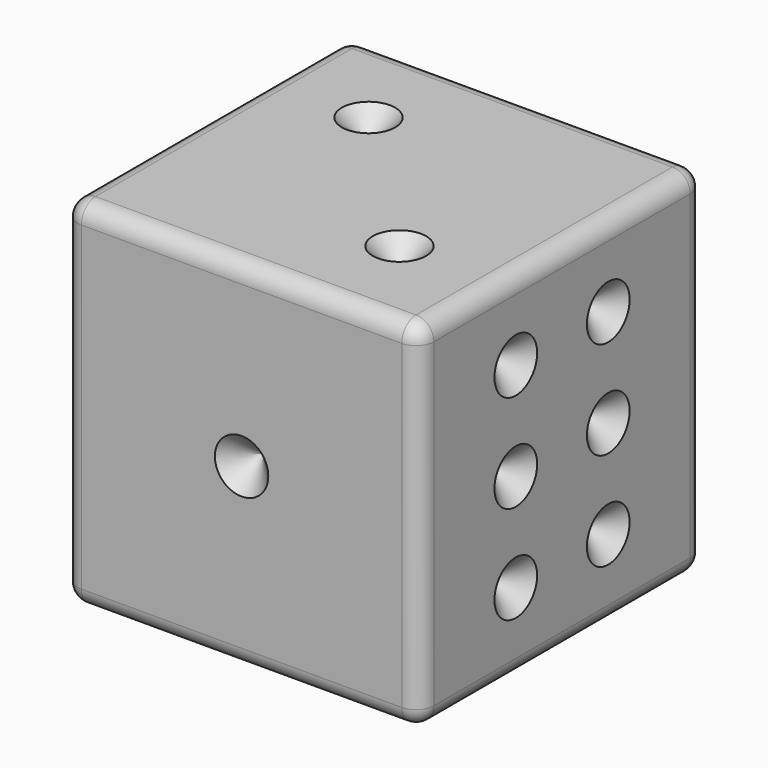
from build123d import *

# Parameters (mm, degrees)
F0_W      = 20
F0_H      = 20
F1_DEPTH  = 20
F2_R      = 1.5
F3_DEPTH  = 1.5
F4_R      = 1.5
F5_DEPTH  = 1.5
F6_SIZE   = 1.49999
F7_SIZE   = 1.49999
F8_R      = 1.5
F9_DEPTH  = 1.5
F10_SIZE  = 1.49999
F11_R     = 1.5
F12_DEPTH = 1.5
F13_SIZE  = 1.49999
F14_R     = 1.5
F15_DEPTH = 1.5
F16_SIZE  = 1.49999
F17_R     = 1.5
F18_DEPTH = 1.5
F19_SIZE  = 1.49999
F20_R     = 1


# Not quite as in the source:
# - a fillet or chamfer is up to 0.001 mm smaller than in the source, because OpenCascade refuses the exact size


with BuildPart() as f1:
    # F0 (on Top) → F1 (new body)
    with BuildSketch(Plane.XY):
        with Locations((10, 10)):
            Rectangle(F0_W, F0_H)
    extrude(amount=F1_DEPTH)

    # F2 (on face) → F3 (cut)
    with BuildSketch(Plane.XZ):
        with Locations((10, 10)):
            Circle(F2_R)
    extrude(amount=-F3_DEPTH, mode=Mode.SUBTRACT)

    # F4 (on face) → F5 (cut)
    with BuildSketch(Plane.XY.offset(20)):
        with Locations((5.6568542495, 14.3431457505)):
            Circle(F4_R)
        with Locations((14.3431457505, 5.6568542495)):
            Circle(F4_R)
    extrude(amount=-F5_DEPTH, mode=Mode.SUBTRACT)

    # F6 (size 1.5 in the source; OpenCascade refuses exactly that, so slightly less here)
    f6_edges = [f1.edges().sort_by_distance(p)[0] for p in [
        (12.843146, 5.656854, 18.5),
        (4.156854, 14.343146, 18.5),
    ]]
    chamfer(f6_edges, length=F6_SIZE)

    # F7 (size 1.5 in the source; OpenCascade refuses exactly that, so slightly less here)
    f7_edges = [f1.edges().sort_by_distance(p)[0] for p in [
        (8.5, 1.5, 10),
    ]]
    chamfer(f7_edges, length=F7_SIZE)

    # F8 (on face) → F9 (cut)
    with BuildSketch(Plane(origin=(0, 20, 0), x_dir=(-1, 0, 0), z_dir=(0, 1, 0))):
        with Locations((-16.1109127035, 16.1109127035)):
            Circle(F8_R)
        with Locations((-10, 10)):
            Circle(F8_R)
        with Locations((-3.8890872965, 3.8890872965)):
            Circle(F8_R)
    extrude(amount=-F9_DEPTH, mode=Mode.SUBTRACT)

    # F10 (size 1.5 in the source; OpenCascade refuses exactly that, so slightly less here)
    f10_edges = [f1.edges().sort_by_distance(p)[0] for p in [
        (17.610913, 18.5, 16.110913),
        (11.5, 18.5, 10),
        (5.389087, 18.5, 3.889087),
    ]]
    chamfer(f10_edges, length=F10_SIZE)

    # F11 (on face) → F12 (cut)
    with BuildSketch(Plane(origin=(0, 0, 0), x_dir=(1, 0, 0), z_dir=(0, 0, -1))):
        with Locations((5.6568542495, -5.6568542495)):
            Circle(F11_R)
        with Locations((14.3431457505, -5.6568542495)):
            Circle(F11_R)
        with Locations((14.3431457505, -14.3431457505)):
            Circle(F11_R)
        with Locations((5.6568542495, -14.3431457505)):
            Circle(F11_R)
    extrude(amount=-F12_DEPTH, mode=Mode.SUBTRACT)

    # F13 (size 1.5 in the source; OpenCascade refuses exactly that, so slightly less here)
    f13_edges = [f1.edges().sort_by_distance(p)[0] for p in [
        (4.156854, 14.343146, 1.5),
        (4.156854, 5.656854, 1.5),
        (12.843146, 5.656854, 1.5),
        (12.843146, 14.343146, 1.5),
    ]]
    chamfer(f13_edges, length=F13_SIZE)

    # F14 (on face) → F15 (cut)
    with BuildSketch(Plane(origin=(0, 0, 0), x_dir=(0, -1, 0), z_dir=(-1, 0, 0))):
        with Locations((-16.1109127035, 16.1109127035)):
            Circle(F14_R)
        with Locations((-3.8890872965, 16.1109127035)):
            Circle(F14_R)
        with Locations((-10, 10)):
            Circle(F14_R)
        with Locations((-16.1109127035, 3.8890872965)):
            Circle(F14_R)
        with Locations((-3.8890872965, 3.8890872965)):
            Circle(F14_R)
    extrude(amount=-F15_DEPTH, mode=Mode.SUBTRACT)

    # F16 (size 1.5 in the source; OpenCascade refuses exactly that, so slightly less here)
    f16_edges = [f1.edges().sort_by_distance(p)[0] for p in [
        (1.5, 17.610913, 16.110913),
        (1.5, 5.389087, 16.110913),
        (1.5, 11.5, 10),
        (1.5, 5.389087, 3.889087),
        (1.5, 17.610913, 3.889087),
    ]]
    chamfer(f16_edges, length=F16_SIZE)

    # F17 (on face) → F18 (cut)
    with BuildSketch(Plane.YZ.offset(20)):
        with Locations((6.7543126643, 15.5)):
            Circle(F17_R)
        with Locations((13.246, 4.5)):
            Circle(F17_R)
        with Locations((6.7543126643, 4.5)):
            Circle(F17_R)
        with Locations((13.246, 15.5)):
            Circle(F17_R)
        with Locations((13.246, 10)):
            Circle(F17_R)
        with Locations((6.7543126643, 10)):
            Circle(F17_R)
    extrude(amount=-F18_DEPTH, mode=Mode.SUBTRACT)

    # F19 (size 1.5 in the source; OpenCascade refuses exactly that, so slightly less here)
    f19_edges = [f1.edges().sort_by_distance(p)[0] for p in [
        (18.5, 5.254313, 15.5),
        (18.5, 11.746, 15.5),
        (18.5, 5.254313, 10),
        (18.5, 11.746, 10),
        (18.5, 11.746, 4.5),
        (18.5, 5.254313, 4.5),
    ]]
    chamfer(f19_edges, length=F19_SIZE)

    # F20
    f20_edges = [f1.edges().sort_by_distance(p)[0] for p in [
        (10, 20, 20),
        (20, 10, 20),
        (0, 10, 20),
        (10, 0, 20),
        (0, 20, 10),
        (0, 10, 0),
        (10, 20, 0),
        (20, 20, 10),
        (0, 0, 10),
        (10, 0, 0),
        (20, 0, 10),
        (20, 10, 0),
    ]]
    fillet(f20_edges, radius=F20_R)


solid = f1.part
